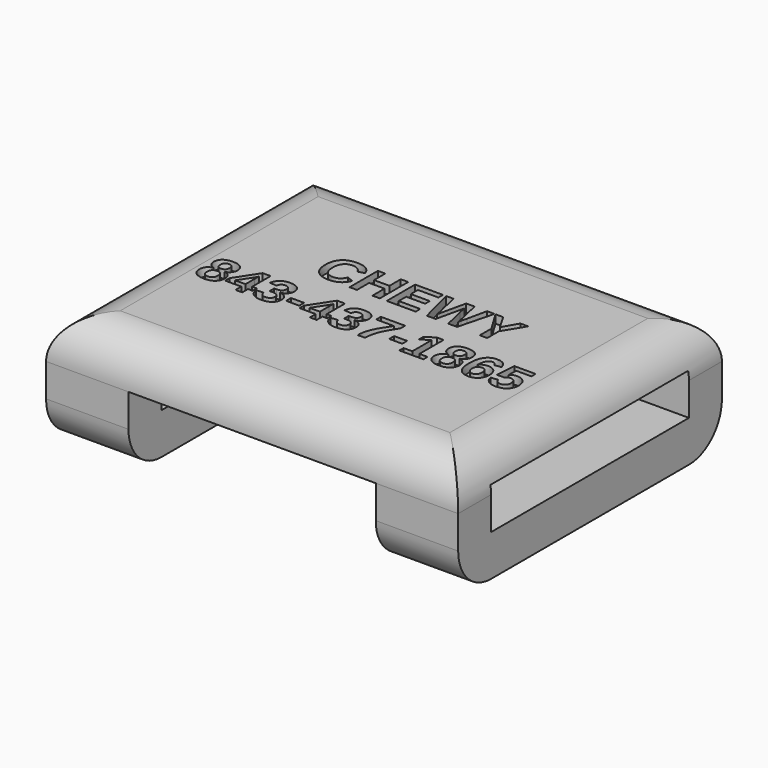
from build123d import *

# Parameters (mm, degrees)
F0_W         = 50
F0_H         = 40
F1_DEPTH     = 14
F2_W         = 30
F2_H         = 5
F3_DEPTH     = 50
F4_W         = 30
F4_H         = 18
F5_DEPTH     = 40
F6_T1_DEPTH  = 75
F6_T3_DEPTH  = 65
F6_T5_DEPTH  = 35
F6_T7_DEPTH  = 35
F8_TEXT_SIZE = 6.25
F9_DEPTH     = 1


# Not quite as in the source:
# - a fillet or chamfer that OpenCascade refuses, or shapes differently, is made with other operations: its cross-section is extruded or revolved along the edge and cut away or added
# - Text() gives the source's letters only with a copy of the font that has no kerning and outlines rounded to 1/6400 em; it was checked with that copy


with BuildPart() as f1:
    # F0 (on Top) → F1 (new body)
    with BuildSketch(Plane.XY):
        Rectangle(F0_W, F0_H)
    extrude(amount=F1_DEPTH)

    # F2 (on face) → F3 (cut)
    with BuildSketch(Plane(origin=(-25, 0, 0), x_dir=(0, -1, 0), z_dir=(-1, 0, 0))):
        with Locations((0, 7.5)):
            Rectangle(F2_W, F2_H)
    extrude(amount=-F3_DEPTH, mode=Mode.SUBTRACT)

    # F4 (on face) → F5 (cut, through all)
    with BuildSketch(Plane.XZ.offset(20)):
        Rectangle(F4_W, F4_H)
    extrude(amount=-F5_DEPTH, mode=Mode.SUBTRACT)

    # F6: fillet of radius 5 on 8 edges, made by hand

    # F6_s2 → F6_t1 (cut)
    with BuildSketch(Plane.YZ.offset(-37.5)):
        with BuildLine():
            ThreePointArc((20, 9), (18.5355339059, 12.5355339059), (15, 14))
            Line((15, 14), (20, 14))
            Line((20, 14), (20, 9))
        make_face()
        with BuildLine():
            ThreePointArc((-15, 14), (-18.5355339059, 12.5355339059), (-20, 9))
            Line((-20, 9), (-20, 14))
            Line((-20, 14), (-15, 14))
        make_face()
    extrude(amount=F6_T1_DEPTH, mode=Mode.SUBTRACT)

    # F6_s4 → F6_t3 (cut)
    with BuildSketch(Plane.XZ.offset(-32.5)):
        with BuildLine():
            ThreePointArc((-25, 9), (-23.5355339059, 12.5355339059), (-20, 14))
            Line((-20, 14), (-25, 14))
            Line((-25, 14), (-25, 9))
        make_face()
        with BuildLine():
            ThreePointArc((20, 14), (23.5355339059, 12.5355339059), (25, 9))
            Line((25, 9), (25, 14))
            Line((25, 14), (20, 14))
        make_face()
    extrude(amount=F6_T3_DEPTH, mode=Mode.SUBTRACT)

    # F6_s6 → F6_t5 (cut)
    with BuildSketch(Plane.YZ.offset(-37.5)):
        with BuildLine():
            ThreePointArc((20, 5), (18.5355339059, 1.4644660941), (15, 0))
            Line((15, 0), (20, 0))
            Line((20, 0), (20, 5))
        make_face()
        with BuildLine():
            ThreePointArc((-15, 0), (-18.5355339059, 1.4644660941), (-20, 5))
            Line((-20, 5), (-20, 0))
            Line((-20, 0), (-15, 0))
        make_face()
    extrude(amount=F6_T5_DEPTH, mode=Mode.SUBTRACT)

    # F6_s8 → F6_t7 (cut)
    with BuildSketch(Plane.YZ.offset(2.5)):
        with BuildLine():
            ThreePointArc((20, 5), (18.5355339059, 1.4644660941), (15, 0))
            Line((15, 0), (20, 0))
            Line((20, 0), (20, 5))
        make_face()
        with BuildLine():
            ThreePointArc((-15, 0), (-18.5355339059, 1.4644660941), (-20, 5))
            Line((-20, 5), (-20, 0))
            Line((-20, 0), (-15, 0))
        make_face()
    extrude(amount=F6_T7_DEPTH, mode=Mode.SUBTRACT)

    # F8 (on offset) → F9 (cut)
    with BuildSketch(Plane.XY.offset(14)):
        with Locations((-10.9939306212, 2.3501984853)):
            Text('CHEWY', F8_TEXT_SIZE, font='Arimo', font_style=FontStyle.BOLD, text_align=(TextAlign.LEFT, TextAlign.BOTTOM))
        with Locations((-19.6755712462, -4.8373015147)):
            Text('843-437-1865', F8_TEXT_SIZE, font='Arimo', font_style=FontStyle.BOLD, text_align=(TextAlign.LEFT, TextAlign.BOTTOM))
    extrude(amount=-F9_DEPTH, mode=Mode.SUBTRACT)


solid = f1.part
